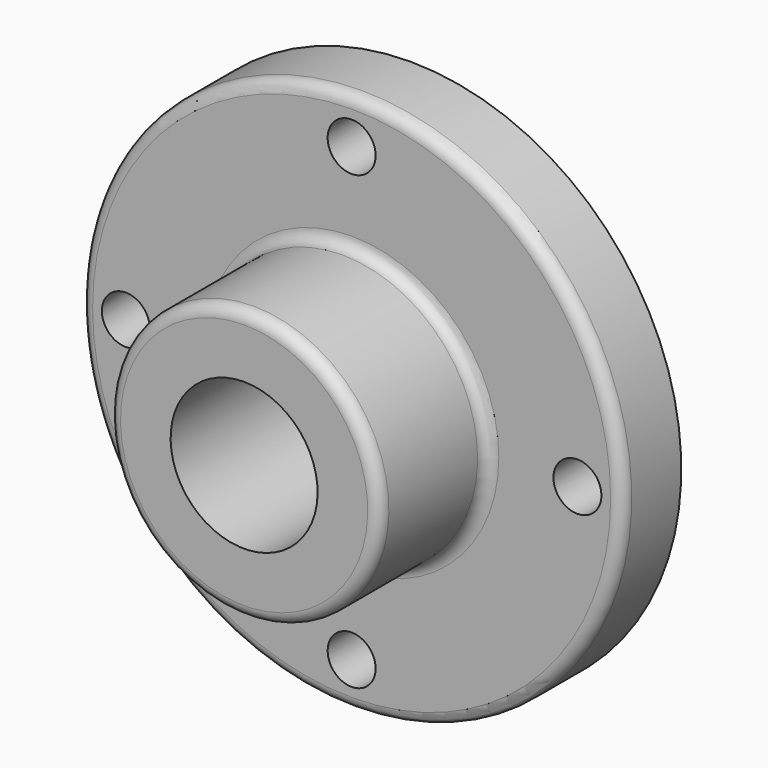
from build123d import *

# Parameters (mm, degrees)
F2_R            = 6.2084574244
F3_DEPTH        = 53.848
F3_COPIES_COUNT = 4
F6_W            = 53.848
F6_H            = 19.0246
F8_R            = 3.048


# Not quite as in the source:
# - a pattern or mirror of a feature is missing from the dataset's text; its kind, count and spacing are read off the source's solid


with BuildPart() as f1:
    # F0 (on Right) → F1 (revolve)
    with BuildSketch(Plane.YZ):
        with BuildLine():
            Line((-19.05, 0), (0, 0))
            Line((0, 0), (0, 70.104))
            Line((0, 70.104), (-16.002, 70.104))
            ThreePointArc((-16.002, 70.104), (-18.1572614691, 69.2112614691), (-19.05, 67.056))
            Line((-19.05, 67.056), (-19.05, 0))
        make_face()
    revolve(axis=Axis((0, -9.525, 0), (0, -1, 0)))

    # F2 (on Front) → F3 (cut)
    with BuildSketch(Plane.XZ):
        with Locations((0, 58.4511086345)):
            Circle(F2_R)
    f3 = extrude(amount=F3_DEPTH, mode=Mode.SUBTRACT)

    # F3_copies: F3 ×4 about axis
    f3_copies_axis = Axis((0, 0, 0), (0, 1, 0))
    for i in range(1, F3_COPIES_COUNT):
        add(f3.rotate(f3_copies_axis, i * 360 / F3_COPIES_COUNT), mode=Mode.SUBTRACT)

    # F4 (on Right) → F5 (revolve)
    with BuildSketch(Plane.YZ):
        with BuildLine():
            Line((-53.848, 0), (0, 0))
            Line((0, 0), (0, 35.052))
            Line((0, 35.052), (-50.8, 35.052))
            ThreePointArc((-50.8, 35.052), (-52.9552614691, 34.1592614691), (-53.848, 32.004))
            Line((-53.848, 32.004), (-53.848, 0))
        make_face()
    revolve(axis=Axis((0, -26.924, 0), (0, -1, 0)))

    # F6 (on Right) → F7 (revolve, cut)
    with BuildSketch(Plane.YZ):
        with Locations((-26.924, 9.5123)):
            Rectangle(F6_W, F6_H)
    revolve(axis=Axis((0, -26.924, 0), (0, -1, 0)), mode=Mode.SUBTRACT)

    # F8
    f8_edges = [f1.edges().sort_by_distance(p)[0] for p in [
        (0, -19.05, -35.052),
    ]]
    fillet(f8_edges, radius=F8_R)


solid = f1.part
